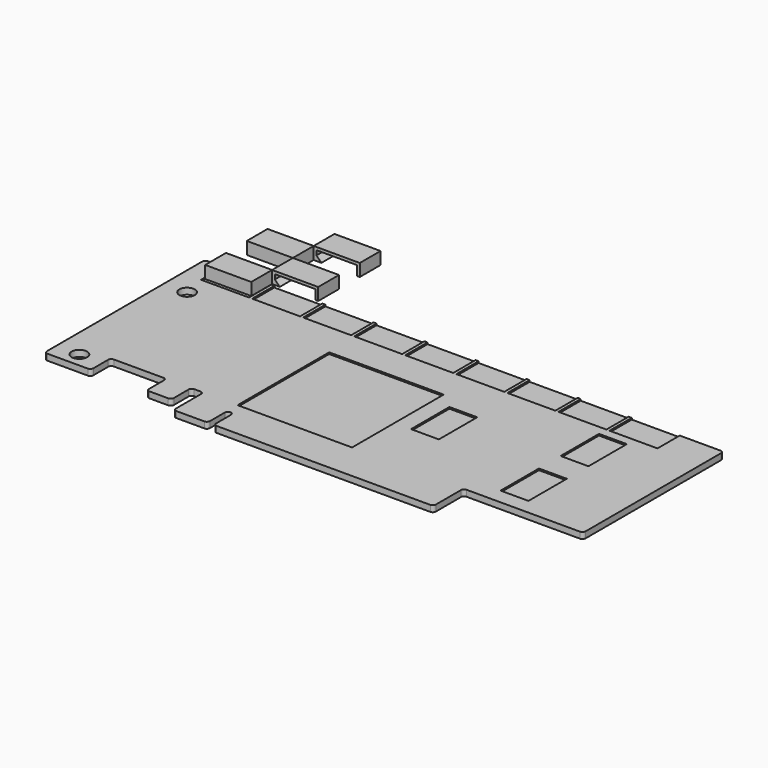
from build123d import *

# Parameters (mm, degrees)
F0_R      = 2.5
F1_DEPTH  = 2
F3_R      = 0.99999
F2_W      = 15.5
F2_H      = 9
F2_W_2    = 9
F2_H_2    = 15.5
F2_W_3    = 37
F2_H_3    = 37
F4_DEPTH  = 0.5
F6_W      = 14.9
F6_H      = 8.4
F7_DEPTH  = 4
F9_DEPTH  = 6
F11_ANGLE = 180
F12_ANGLE = 180
F13_ANGLE = 180


# Not quite as in the source:
# - a fillet or chamfer is up to 0.001 mm smaller than in the source, because OpenCascade refuses the exact size


with BuildPart() as f1:
    # F0 (on Top) → F1 (new body)
    with BuildSketch(Plane.XY):
        Polygon((83.825, -24.3705166107), (83.825, 32.3705166107), (-83.825, 32.3705166107), (-83.825, -32.3705166107), (-68.825, -32.3705166107), (-68.825, -24.3705166107), (-50.825, -24.3705166107), (-50.825, -32.3705166107), (-42.825, -32.3705166107), (-42.825, -24.3705166107), (-38.825, -24.3705166107), (-38.825, -36.5294833893), (-27.825, -36.5294833893), (-27.825, -28.5294833893), (-25.825, -28.5294833893), (-25.825, -36.5294833893), (45.175, -36.5294833893), (45.175, -24.3705166107), align=None)
        with Locations((-76.325, -27.6294833893)):
            Circle(F0_R, mode=Mode.SUBTRACT)
        with Locations((-76.325, 15.8705166107)):
            Circle(F0_R, mode=Mode.SUBTRACT)
    extrude(amount=F1_DEPTH)

    # F3 (radius 1 in the source; OpenCascade refuses exactly that, so slightly less here)
    f3_edges = [f1.edges().sort_by_distance(p)[0] for p in [
        (-83.825, -32.370517, 1),
        (-68.825, -32.370517, 1),
        (-68.825, -24.370517, 1),
        (-50.825, -32.370517, 1),
        (-42.825, -32.370517, 1),
        (-42.825, -24.370517, 1),
        (-38.825, -36.529483, 1),
        (-27.825, -36.529483, 1),
        (-27.825, -28.529483, 1),
        (-25.825, -36.529483, 1),
        (83.825, -24.370517, 1),
        (45.175, -24.370517, 1),
        (45.175, -36.529483, 1),
        (83.825, 32.370517, 1),
        (-83.825, 32.370517, 1),
        (-50.825, -24.370517, 1),
        (-38.825, -24.370517, 1),
        (-25.825, -28.529483, 1),
    ]]
    fillet(f3_edges, radius=F3_R)

    # F2 (on face) → F4 (cut)
    with BuildSketch(Plane.XY.offset(2)):
        with Locations((-70.075, 27.8705166107)):
            Rectangle(F2_W, F2_H)
        with Locations((-53.575, 27.8705166107)):
            Rectangle(F2_W, F2_H)
        with Locations((-37.075, 27.8705166107)):
            Rectangle(F2_W, F2_H)
        with Locations((-20.575, 27.8705166107)):
            Rectangle(F2_W, F2_H)
        with Locations((-4.075, 27.8705166107)):
            Rectangle(F2_W, F2_H)
        with Locations((12.425, 27.8705166107)):
            Rectangle(F2_W, F2_H)
        with Locations((28.925, 27.8705166107)):
            Rectangle(F2_W, F2_H)
        with Locations((45.425, 27.8705166107)):
            Rectangle(F2_W, F2_H)
        with Locations((61.925, 27.8705166107)):
            Rectangle(F2_W, F2_H)
        with Locations((57.675, 12.6205166107)):
            Rectangle(F2_W_2, F2_H_2)
        with Locations((57.675, -11.6205166107)):
            Rectangle(F2_W_2, F2_H_2)
        with Locations((19.0305227488, 0.5)):
            Rectangle(F2_W_2, F2_H_2)
        with Locations((-9.325, -5.8705166107)):
            Rectangle(F2_W_3, F2_H_3)
    extrude(amount=-F4_DEPTH, mode=Mode.SUBTRACT)


with BuildPart() as f7:
    # F6 (on offset) → F7 (new body)
    with BuildSketch(Plane.XY.offset(1.8)):
        with Locations((-70.075, 27.8705166107)):
            Rectangle(F6_W, F6_H)
    extrude(amount=F7_DEPTH)

    # F8 (on face) → F9 (cut)
    with BuildSketch(Plane(origin=(0, 32.0705166107, 0), x_dir=(-1, 0, 0), z_dir=(0, 1, 0))):
        Polygon((65.125, 1.8), (76.625, 1.8), (76.625, 4.9), (63.525, 4.9), (63.525, 3.4), align=None)
    extrude(amount=-F9_DEPTH, mode=Mode.SUBTRACT)


with BuildPart() as f7_1:
    # F10: moved
    add(f7.part.moved(Location((0, 1, 0))))


with BuildPart() as f11_1:
    # F11: copy of F7
    add(f7_1.part.rotate(Axis((-62.625, 33.0705166107, 3.8), (0, 0, -1)), F11_ANGLE))


with BuildPart() as f12_1:
    # F12: copy of F11_1
    add(f11_1.part.rotate(Axis((-62.625, 41.4705166107, 3.8), (0, 0, 1)), F12_ANGLE))


with BuildPart() as f13_1:
    # F13: copy of F12_1
    add(f12_1.part.rotate(Axis((-62.625, 49.8705166107, 3.8), (0, 0, -1)), F13_ANGLE))


solid = Compound([f1.part, f7_1.part, f11_1.part, f12_1.part, f13_1.part])
